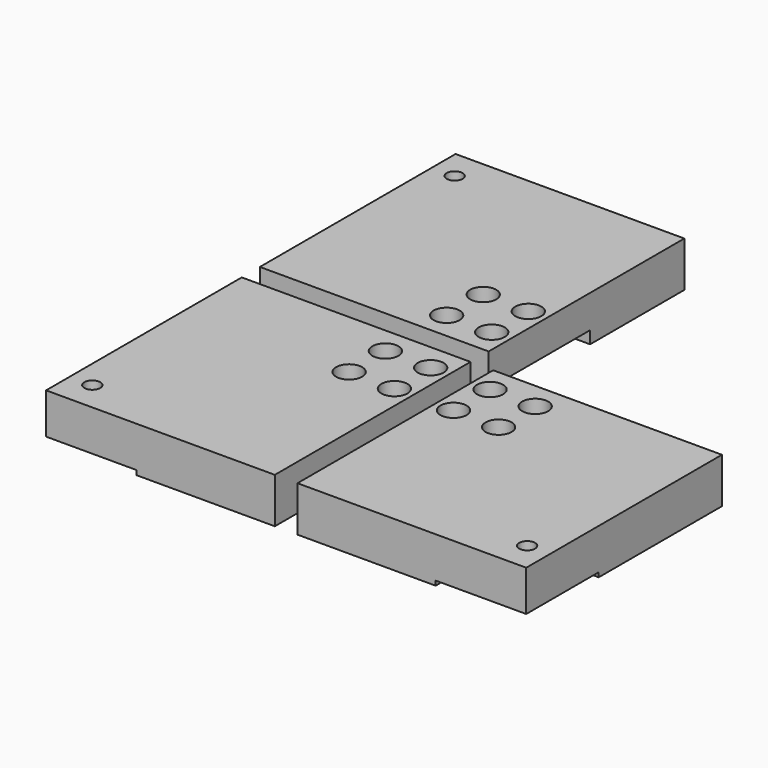
from build123d import *

# Parameters (mm, degrees)
F0_W      = 50.5
F0_H      = 54
F1_DEPTH  = 5
F2_R      = 1.75
F3_DEPTH  = 10
F4_R      = 2.875
F5_DEPTH  = 10
F6_W      = 26.5
F6_H      = 28
F6_R      = 2.875
F7_DEPTH  = 2.75
F8_W      = 20
F8_H      = 20
F8_R      = 1.75
F9_DEPTH  = 1
F10_R     = 4.25
F10_R_2   = 1.75
F11_DEPTH = 3


# Not quite as in the source:
# - a feature names something its author has since deleted; it is built from what else it names


with BuildPart() as f1:
    # F0 (on Top) → F1 (new body, symmetric)
    with BuildSketch(Plane.XY):
        with Locations((-27.75, 29.5)):
            Rectangle(F0_W, F0_H)
    extrude(amount=F1_DEPTH, both=True)


with BuildPart() as f1b:
    # F0 (on Top) → F1, piece 2 (new body, symmetric)
    with BuildSketch(Plane.XY):
        with Locations((-27.75, -29.5)):
            Rectangle(F0_W, F0_H)
    extrude(amount=F1_DEPTH, both=True)


with BuildPart() as f1c:
    # F0 (on Top) → F1, piece 3 (new body, symmetric)
    with BuildSketch(Plane.XY):
        with Locations((27.75, -29.5)):
            Rectangle(F0_W, F0_H)
    extrude(amount=F1_DEPTH, both=True)


with BuildPart() as f3_tool:
    # F2 (on face) → F3 (new body)
    with BuildSketch(Plane.XY.offset(5)):
        with Locations((-48, 50)):
            Circle(F2_R)
        with Locations((-48, -50)):
            Circle(F2_R)
        with Locations((48, -50)):
            Circle(F2_R)
    extrude(amount=-F3_DEPTH)


with BuildPart() as f1_1:
    add(f1.part)

    # F3: cut by f3_tool
    add(f3_tool.part, mode=Mode.SUBTRACT)


with BuildPart() as f1b_1:
    add(f1b.part)

    # F3: cut by f3_tool
    add(f3_tool.part, mode=Mode.SUBTRACT)


with BuildPart() as f1c_1:
    add(f1c.part)

    # F3: cut by f3_tool
    add(f3_tool.part, mode=Mode.SUBTRACT)


with BuildPart() as f5_tool:
    # F4 (on face) → F5 (new body)
    with BuildSketch(Plane.XY.offset(5)):
        with Locations((-6.5001370548, 18.4476446966)):
            Circle(F4_R)
        with Locations((-16.5, 18.5)):
            Circle(F4_R)
        with Locations((-16.5769208012, 8.5002958449)):
            Circle(F4_R)
        with Locations((-6.577057856, 8.4479405415)):
            Circle(F4_R)
        with Locations((-6.5, -8.5)):
            Circle(F4_R)
        with Locations((-16.5, -8.5)):
            Circle(F4_R)
        with Locations((-16.5, -18.5)):
            Circle(F4_R)
        with Locations((-6.5, -18.5)):
            Circle(F4_R)
        with Locations((6.5001429807, -18.4465248288)):
            Circle(F4_R)
        with Locations((6.5764766346, -8.4468161744)):
            Circle(F4_R)
        with Locations((16.5763336539, -8.5002913456)):
            Circle(F4_R)
        with Locations((16.5, -18.5)):
            Circle(F4_R)
    extrude(amount=-F5_DEPTH)


with BuildPart() as f1_2:
    add(f1_1.part)

    # F5: cut by f5_tool
    add(f5_tool.part, mode=Mode.SUBTRACT)


with BuildPart() as f1b_2:
    add(f1b_1.part)

    # F5: cut by f5_tool
    add(f5_tool.part, mode=Mode.SUBTRACT)


with BuildPart() as f1c_2:
    add(f1c_1.part)

    # F5: cut by f5_tool
    add(f5_tool.part, mode=Mode.SUBTRACT)


with BuildPart() as f7_tool:
    # F6 (on face) → F7 (new body)
    with BuildSketch(Plane(origin=(0, 0, -5), x_dir=(1, 0, 0), z_dir=(0, 0, -1))):
        with Locations((15.75, 16.5)):
            Rectangle(F6_W, F6_H)
        with Locations((-15.75, -16.5)):
            Rectangle(F6_W, F6_H)
        with Locations((-15.75, 16.5)):
            Rectangle(F6_W, F6_H)
        with Locations((-16.5, 8.5)):
            Circle(F6_R, mode=Mode.SUBTRACT)
        with Locations((-6.5, 8.5)):
            Circle(F6_R, mode=Mode.SUBTRACT)
        with Locations((-16.5, 18.5)):
            Circle(F6_R, mode=Mode.SUBTRACT)
        with Locations((-6.5, 18.5)):
            Circle(F6_R, mode=Mode.SUBTRACT)
    extrude(amount=-F7_DEPTH)


with BuildPart() as f1_3:
    add(f1_2.part)

    # F7: cut by f7_tool
    add(f7_tool.part, mode=Mode.SUBTRACT)


with BuildPart() as f1b_3:
    add(f1b_2.part)

    # F7: cut by f7_tool
    add(f7_tool.part, mode=Mode.SUBTRACT)


with BuildPart() as f1c_3:
    add(f1c_2.part)

    # F7: cut by f7_tool
    add(f7_tool.part, mode=Mode.SUBTRACT)


with BuildPart() as f9_tool:
    # F8 (on face) → F9 (new body)
    with BuildSketch(Plane(origin=(0, 0, -5), x_dir=(1, 0, 0), z_dir=(0, 0, -1))):
        with Locations((-43, -46.5)):
            Rectangle(F8_W, F8_H)
        with Locations((-48, -50)):
            Circle(F8_R, mode=Mode.SUBTRACT)
        with Locations((-43, 46.5)):
            Rectangle(F8_W, F8_H)
        with Locations((43, 46.5)):
            Rectangle(F8_W, F8_H)
    extrude(amount=-F9_DEPTH)


with BuildPart() as f1_4:
    add(f1_3.part)

    # F9: cut by f9_tool
    add(f9_tool.part, mode=Mode.SUBTRACT)


with BuildPart() as f1b_4:
    add(f1b_3.part)

    # F9: cut by f9_tool
    add(f9_tool.part, mode=Mode.SUBTRACT)


with BuildPart() as f1c_4:
    add(f1c_3.part)

    # F9: cut by f9_tool
    add(f9_tool.part, mode=Mode.SUBTRACT)


with BuildPart() as f11_tool:
    # F10 (on face) → F11 (new body)
    with BuildSketch(Plane(origin=(0, 0, -4), x_dir=(1, 0, 0), z_dir=(0, 0, -1))):
        with Locations((-48, 50)):
            Circle(F10_R)
        with Locations((-48, 50)):
            Circle(F10_R_2, mode=Mode.SUBTRACT)
        with Locations((48, 50)):
            Circle(F10_R)
        with Locations((-48, -50)):
            Circle(F10_R)
    extrude(amount=-F11_DEPTH)


with BuildPart() as f1_5:
    add(f1_4.part)

    # F11: cut by f11_tool
    add(f11_tool.part, mode=Mode.SUBTRACT)


with BuildPart() as f1b_5:
    add(f1b_4.part)

    # F11: cut by f11_tool
    add(f11_tool.part, mode=Mode.SUBTRACT)


with BuildPart() as f1c_5:
    add(f1c_4.part)

    # F11: cut by f11_tool
    add(f11_tool.part, mode=Mode.SUBTRACT)


solid = Compound([f1_5.part, f1b_5.part, f1c_5.part])
